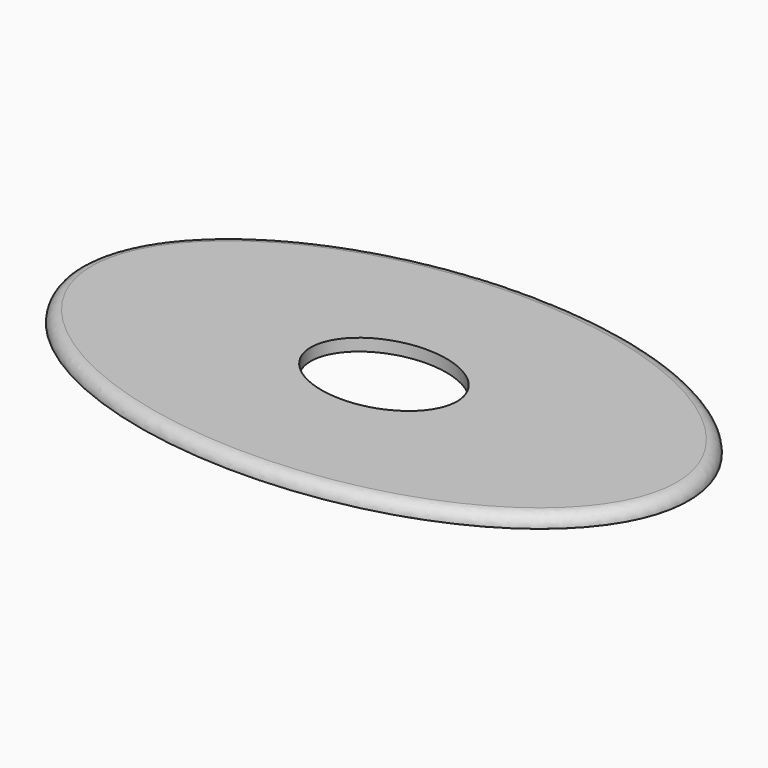
from build123d import *

# Parameters (mm, degrees)
F1_DEPTH = 5
F2_R     = 4.999
F4_DEPTH = 25


# Not quite as in the source:
# - a fillet or chamfer is up to 0.001 mm smaller than in the source, because OpenCascade refuses the exact size


with BuildPart() as f1:
    # F0 (on Top) → F1 (new body)
    with BuildSketch(Plane.XY):
        with BuildLine():
            add(Edge.make_bspline(
                [(-125, 0), (-125, -129.903811), (62.5, -64.951905), (250, 0), (62.5, 64.951905), (-125, 129.903811), (-125, 0)],
                knots=[0, 0, 0, 2.094395, 2.094395, 4.18879, 4.18879, 6.283185, 6.283185, 6.283185], degree=2, weights=[1, 0.5, 1, 0.5, 1, 0.5, 1]))
        make_face()
    extrude(amount=F1_DEPTH)

    # F2 (radius 5 in the source; OpenCascade refuses exactly that, so slightly less here)
    f2_edges = [f1.edges().sort_by_distance(p)[0] for p in [
        (125, -1e-06, 5),
    ]]
    fillet(f2_edges, radius=F2_R)

    # F3 (on face) → F4 (cut)
    with BuildSketch(Plane.XY.offset(5)):
        with BuildLine():
            add(Edge.make_bspline(
                [(-30, 0), (-30, -38.105118), (15, -19.052559), (60, 0), (15, 19.052559), (-30, 38.105118), (-30, 0)],
                knots=[0, 0, 0, 2.094395, 2.094395, 4.18879, 4.18879, 6.283185, 6.283185, 6.283185], degree=2, weights=[1, 0.5, 1, 0.5, 1, 0.5, 1]))
        make_face()
    extrude(amount=-F4_DEPTH, mode=Mode.SUBTRACT)


solid = f1.part
